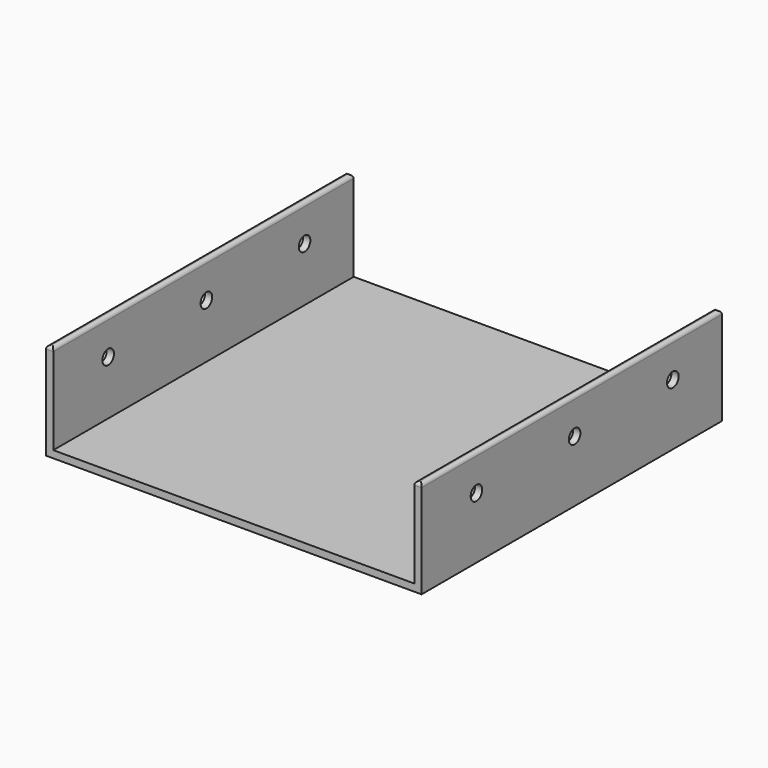
from build123d import *

# Parameters (mm, degrees)
F0_W     = 104
F0_H     = 104
F1_DEPTH = 2
F2_W     = 2
F2_H     = 104
F3_DEPTH = 25
F4_W     = 2
F4_H     = 104
F5_DEPTH = 25
F6_R     = 0.99999
F7_R     = 0.99999
F9_D     = 4
F11_D    = 4
F13_D    = 4


# Not quite as in the source:
# - a fillet or chamfer is up to 0.001 mm smaller than in the source, because OpenCascade refuses the exact size


with BuildPart() as f1:
    # F0 (on Top) → F1 (new body)
    with BuildSketch(Plane.XY):
        Rectangle(F0_W, F0_H)
    extrude(amount=F1_DEPTH)

    # F2 (on face) → F3 (join)
    with BuildSketch(Plane.XY.offset(2)):
        with Locations((-51, 0)):
            Rectangle(F2_W, F2_H)
    extrude(amount=F3_DEPTH)

    # F4 (on face) → F5 (join)
    with BuildSketch(Plane.XY.offset(2)):
        with Locations((51, 0)):
            Rectangle(F4_W, F4_H)
    extrude(amount=F5_DEPTH)

    # F6 (radius 1 in the source; OpenCascade refuses exactly that, so slightly less here)
    f6_edges = [f1.edges().sort_by_distance(p)[0] for p in [
        (52, 0, 27),
        (51, 52, 27),
        (50, 0, 27),
        (51, -52, 27),
    ]]
    fillet(f6_edges, radius=F6_R)

    # F7 (radius 1 in the source; OpenCascade refuses exactly that, so slightly less here)
    f7_edges = [f1.edges().sort_by_distance(p)[0] for p in [
        (-51, 52, 27),
        (-52, 0, 27),
        (-51, -52, 27),
        (-50, 0, 27),
    ]]
    fillet(f7_edges, radius=F7_R)

    # F9 (through all)
    with Locations(Plane.YZ.offset(52)):
        with Locations((-33, 17)):
            Hole(F9_D / 2)

    # F11 (through all)
    with Locations(Plane.YZ.offset(52)):
        with Locations((1, 17)):
            Hole(F11_D / 2)

    # F13 (through all)
    with Locations(Plane.YZ.offset(52)):
        with Locations((35, 17)):
            Hole(F13_D / 2)


solid = f1.part
